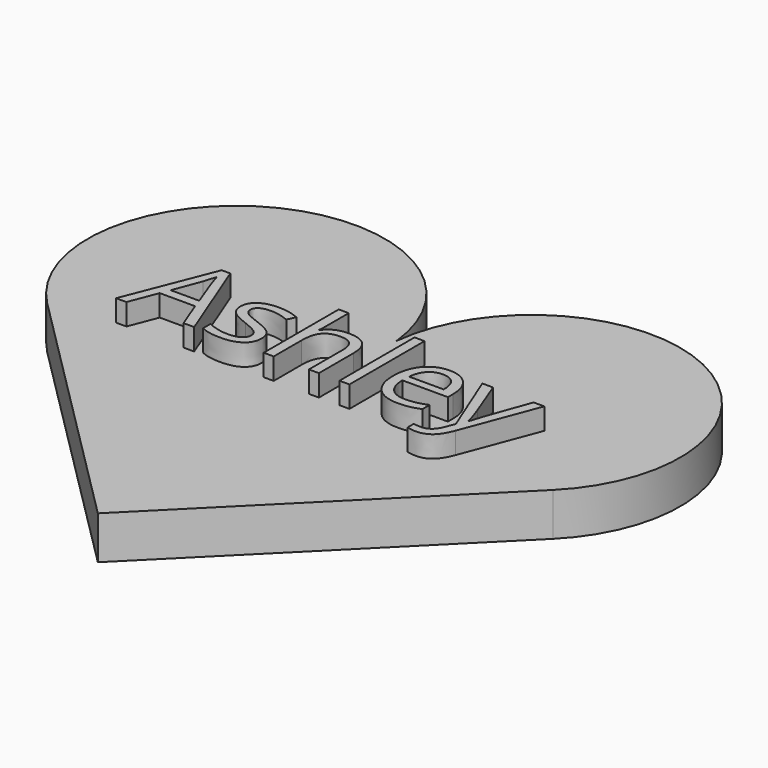
from build123d import *

# Parameters (mm, degrees)
F1_DEPTH     = 5.08
F2_TEXT_SIZE = 14.5610577116
F3_DEPTH     = 7.62


# Not quite as in the source:
# - Text() gives the source's letters only with a copy of the font that has no kerning and outlines rounded to 1/6400 em; it was checked with that copy


with BuildPart() as f1:
    # F0 (on Top) → F1 (new body)
    with BuildSketch(Plane.XY):
        with BuildLine():
            Line((-29.8112200727, 29.802306784), (0, 0))
            Line((0, 0), (29.8099921951, 29.8189077823))
            ThreePointArc((29.8099921951, 29.8189077823), (24.9557565965, 58.0168676622), (0, 44.0204839388))
            ThreePointArc((0, 44.0204839388), (-24.9666383493, 58.0063308041), (-29.8112200727, 29.802306784))
        make_face()
    extrude(amount=F1_DEPTH)

    # F2 (on Top) → F3 (join)
    with BuildSketch(Plane.XY):
        with Locations((-22.4467778171, 30.7445004582)):
            Text('Ashley', F2_TEXT_SIZE, font='Open Sans', text_align=(TextAlign.LEFT, TextAlign.BOTTOM))
    extrude(amount=F3_DEPTH)


solid = f1.part
